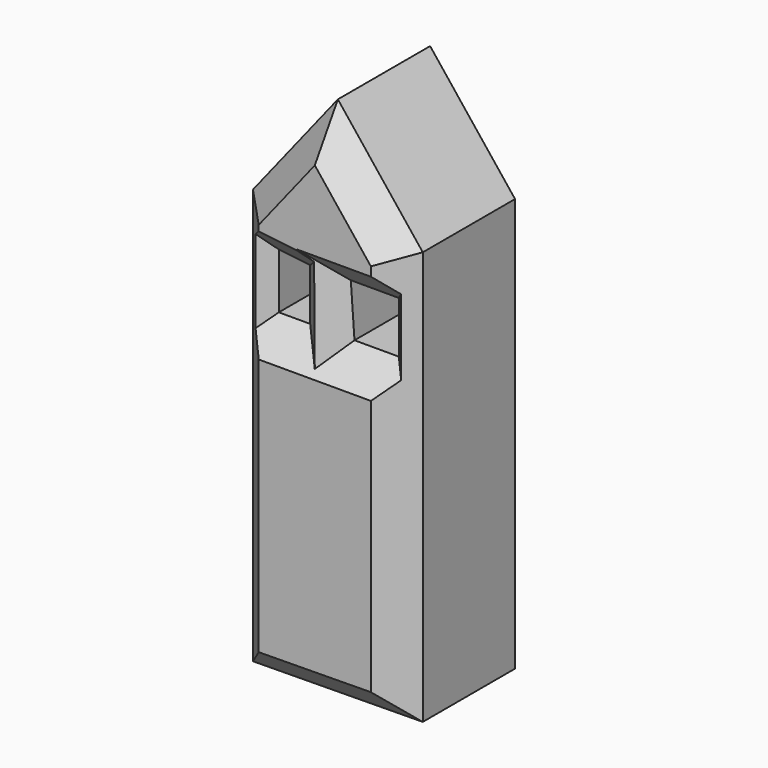
from build123d import *

# Parameters (mm, degrees)
F1_DEPTH      = 25.4
F2_T1_DEPTH   = 5.5291503668
F2_T3_DEPTH   = 9.1068297625
F2_T8_DEPTH   = 98.9829335321
F2_T14_DEPTH  = 50.2051374371
F2_T20_DEPTH  = 50.2051368583
F2_T26_DEPTH  = 99.3081774522
F2_T32_DEPTH  = 56.0525045898
F2_T38_DEPTH  = 22.8214690441
F2_T43_DEPTH  = 31.6955822143
F2_T49_DEPTH  = 22.1709793413
F2_T54_DEPTH  = 35.2583310718
F2_T60_DEPTH  = 21.5204924325
F2_T65_DEPTH  = 20.8700045923
F2_T71_DEPTH  = 98.9829335321
F2_T75_DEPTH  = 56.0525045898
F2_T82_DEPTH  = 98.9829335321
F2_T86_DEPTH  = 50.2051374371
F2_T93_DEPTH  = 50.2051374371
F2_T97_DEPTH  = 50.2051368583
F2_T104_DEPTH = 50.2051368583
F2_T108_DEPTH = 99.3081774522
F2_T115_DEPTH = 99.3081774522
F2_T119_DEPTH = 56.0525045898
F2_T126_DEPTH = 35.885618623
F2_T130_DEPTH = 18.5932999456
F2_T137_DEPTH = 22.8214690441
F2_T141_DEPTH = 31.6955822143
F2_T148_DEPTH = 31.6955822143
F2_T152_DEPTH = 22.1709793413
F2_T159_DEPTH = 35.2351289202
F2_T163_DEPTH = 18.5932999456
F2_T170_DEPTH = 35.2583310718
F2_T174_DEPTH = 20.8700045923
F2_T181_DEPTH = 35.2583310718
F2_T185_DEPTH = 21.5204924325
F2_T192_DEPTH = 34.5846420113
F2_T196_DEPTH = 22.1709793413
F2_T203_DEPTH = 22.1709793413
F2_T207_DEPTH = 33.9341541712
F3_R          = 2.4287646607
F4_DEPTH      = 25.4


# Not quite as in the source:
# - a fillet or chamfer that OpenCascade refuses, or shapes differently, is made with other operations: its cross-section is extruded or revolved along the edge and cut away or added


with BuildPart() as f1:
    # F0 (on Front) → F1 (new body)
    with BuildSketch(Plane.XZ):
        Polygon((-38.8666465878, 36.5899391472), (-38.8666465878, -36.5899391472), (-8.9442087337, -36.2646952271), (-8.9442087337, 36.5899391472), align=None)
        Polygon((-34.3132354319, 19.0267674625), (-34.3132354319, 28.7840869278), (-28.7840850651, 28.133597225), (-28.7840850651, 19.0267674625), align=None, mode=Mode.SUBTRACT)
        Polygon((-20.9782328457, 19.0267674625), (-21.6287206858, 28.133597225), (-13.1723778322, 28.133597225), (-13.1723778322, 19.0267674625), align=None, mode=Mode.SUBTRACT)
        Polygon((-23.9054281265, 55.4540865123), (-38.8666465878, 36.5899391472), (-8.9442087337, 36.5899391472), align=None)
    extrude(amount=F1_DEPTH)

    # F2: chamfer of 5.08 on 13 edges, made by hand

    # F2_s2 → F2_t1 (cut)
    with BuildSketch(Plane.YZ.offset(-34.3132354319)):
        with BuildLine():
            Line((-20.1763159021, 19.1704515604), (-25.5436840979, 13.8030833646))
            Line((-25.5436840979, 13.8030833646), (-25.6452840979, 13.8030833646))
            ThreePointArc((-25.6452840979, 13.8030833646), (-25.5016, 16.4149254135), (-25.5016, 19.0267674625))
            Line((-25.5016, 19.0267674625), (-25.4, 19.1283674625))
            ThreePointArc((-25.4, 19.1283674625), (-22.788157951, 19.1283674625), (-20.1763159021, 19.2720515604))
            Line((-20.1763159021, 19.2720515604), (-20.1763159021, 19.1704515604))
        make_face()
    extrude(amount=F2_T1_DEPTH, mode=Mode.SUBTRACT)

    # F2_s4 → F2_t3 (cut)
    with BuildSketch(Plane.XY.offset(19.0267674625)):
        with BuildLine():
            Line((-13.3160619302, -20.1763159021), (-7.9486937343, -25.5436840979))
            Line((-7.9486937343, -25.5436840979), (-7.9486937343, -25.6452840979))
            ThreePointArc((-7.9486937343, -25.6452840979), (-10.5605357833, -25.5016), (-13.1723778322, -25.5016))
            Line((-13.1723778322, -25.5016), (-13.2739778322, -25.4))
            ThreePointArc((-13.2739778322, -25.4), (-13.2739778322, -22.788157951), (-13.4176619302, -20.1763159021))
            Line((-13.4176619302, -20.1763159021), (-13.3160619302, -20.1763159021))
        make_face()
    extrude(amount=F2_T3_DEPTH, mode=Mode.SUBTRACT)


with BuildPart() as f2_tool6:
    # F2_s7 → F2_t8 (new body)
    with BuildSketch(Plane.XY.offset(-49.328844806)):
        with BuildLine():
            Line((-8.8005246358, -20.1763159021), (-14.1678928317, -25.5436840979))
            Line((-14.1678928317, -25.5436840979), (-14.1678928317, -25.6452840979))
            ThreePointArc((-14.1678928317, -25.6452840979), (-11.5560507827, -25.5016), (-8.9442087337, -25.5016))
            Line((-8.9442087337, -25.5016), (-8.8426087337, -25.4))
            ThreePointArc((-8.8426087337, -25.4), (-8.8426087337, -22.788157951), (-8.6989246358, -20.1763159021))
            Line((-8.6989246358, -20.1763159021), (-8.8005246358, -20.1763159021))
        make_face()
    extrude(amount=F2_T8_DEPTH)

    split(bisect_by=Plane(origin=(0.3930783298, 0, -36.163202967), x_dir=(0, 1, 0), z_dir=(-0.0108689242, 0, 0.9999409315)), keep=Keep.TOP)

    split(bisect_by=Plane(origin=(12.3236563201, 0, 9.7739337144), x_dir=(0, 1, 0), z_dir=(-0.7834976979, 0, -0.6213946873)), keep=Keep.TOP)


with BuildPart() as f1_1:
    add(f1.part)

    # F2_t5: cut F2_tool6
    add(f2_tool6.part, mode=Mode.SUBTRACT)


with BuildPart() as f2_tool12:
    # F2_s13 → F2_t14 (new body)
    with BuildSketch(Plane(origin=(-13.149871912, 0, 16.5802743125), x_dir=(0, 1, 0), z_dir=(-0.6213946873, 0, 0.7834976979))):
        with BuildLine():
            Line((-20.1763159021, -15.8727109385), (-25.5436840979, -10.5053427426))
            Line((-25.5436840979, -10.5053427426), (-25.6452840979, -10.5053427426))
            ThreePointArc((-25.6452840979, -10.5053427426), (-25.5016, -13.1171847916), (-25.5016, -15.7290268405))
            Line((-25.5016, -15.7290268405), (-25.4, -15.8306268405))
            ThreePointArc((-25.4, -15.8306268405), (-22.788157951, -15.8306268405), (-20.1763159021, -15.9743109385))
            Line((-20.1763159021, -15.9743109385), (-20.1763159021, -15.8727109385))
        make_face()
    extrude(amount=F2_T14_DEPTH)

    split(bisect_by=Plane.YZ.offset(-8.9442087337), keep=Keep.BOTTOM)

    split(bisect_by=Plane(origin=(-41.6732420747, 0, 33.0511878754), x_dir=(0, 1, 0), z_dir=(0.7834977168, 0, -0.6213946635)), keep=Keep.TOP)


with BuildPart() as f1_2:
    add(f1_1.part)

    # F2_t11: cut F2_tool12
    add(f2_tool12.part, mode=Mode.SUBTRACT)


with BuildPart() as f2_tool18:
    # F2_s19 → F2_t20 (new body)
    with BuildSketch(Plane(origin=(25.8858067798, 0, 32.6386300033), x_dir=(0, 1, 0), z_dir=(-0.6213946635, 0, -0.7834977168))):
        with BuildLine():
            Line((-20.1763159021, -53.3324058817), (-25.5436840979, -47.9650376858))
            Line((-25.5436840979, -47.9650376858), (-25.6452840979, -47.9650376858))
            ThreePointArc((-25.6452840979, -47.9650376858), (-25.5016, -50.5768797348), (-25.5016, -53.1887217838))
            Line((-25.5016, -53.1887217838), (-25.4, -53.2903217838))
            ThreePointArc((-25.4, -53.2903217838), (-22.788157951, -53.2903217838), (-20.1763159021, -53.4340058817))
            Line((-20.1763159021, -53.4340058817), (-20.1763159021, -53.3324058817))
        make_face()
    extrude(amount=F2_T20_DEPTH)

    split(bisect_by=Plane(origin=(12.3236563201, 0, 9.7739337144), x_dir=(0, 1, 0), z_dir=(-0.7834976979, 0, -0.6213946873)), keep=Keep.TOP)

    split(bisect_by=Plane.YZ.offset(-38.8666465878), keep=Keep.TOP)


with BuildPart() as f1_3:
    add(f1_2.part)

    # F2_t17: cut F2_tool18
    add(f2_tool18.part, mode=Mode.SUBTRACT)


with BuildPart() as f2_tool24:
    # F2_s25 → F2_t26 (new body)
    with BuildSketch(Plane.XY.offset(49.6540887261)):
        with BuildLine():
            Line((-39.0103306858, -20.1763159021), (-33.6429624899, -25.5436840979))
            Line((-33.6429624899, -25.5436840979), (-33.6429624899, -25.6452840979))
            ThreePointArc((-33.6429624899, -25.6452840979), (-36.2548045389, -25.5016), (-38.8666465878, -25.5016))
            Line((-38.8666465878, -25.5016), (-38.9682465878, -25.4))
            ThreePointArc((-38.9682465878, -25.4), (-38.9682465878, -22.788157951), (-39.1119306858, -20.1763159021))
            Line((-39.1119306858, -20.1763159021), (-39.0103306858, -20.1763159021))
        make_face()
    extrude(amount=-F2_T26_DEPTH)

    split(bisect_by=Plane(origin=(-41.6732420747, 0, 33.0511878754), x_dir=(0, 1, 0), z_dir=(0.7834977168, 0, -0.6213946635)), keep=Keep.TOP)

    split(bisect_by=Plane(origin=(0.3930783298, 0, -36.163202967), x_dir=(0, 1, 0), z_dir=(-0.0108689242, 0, 0.9999409315)), keep=Keep.TOP)


with BuildPart() as f1_4:
    add(f1_3.part)

    # F2_t23: cut F2_tool24
    add(f2_tool24.part, mode=Mode.SUBTRACT)


with BuildPart() as f2_tool30:
    # F2_s31 → F2_t32 (new body)
    with BuildSketch(Plane(origin=(-52.3231028168, 0, -0.5687294315), x_dir=(0, 1, 0), z_dir=(0.9999409315, 0, 0.0108689242))):
        with BuildLine():
            Line((-20.1763159021, -36.3090232973), (-25.5436840979, -30.9416551014))
            Line((-25.5436840979, -30.9416551014), (-25.6452840979, -30.9416551014))
            ThreePointArc((-25.6452840979, -30.9416551014), (-25.5016, -33.5534971504), (-25.5016, -36.1653391994))
            Line((-25.5016, -36.1653391994), (-25.4, -36.2669391994))
            ThreePointArc((-25.4, -36.2669391994), (-22.788157951, -36.2669391994), (-20.1763159021, -36.4106232973))
            Line((-20.1763159021, -36.4106232973), (-20.1763159021, -36.3090232973))
        make_face()
    extrude(amount=F2_T32_DEPTH)

    split(bisect_by=Plane.YZ.offset(-8.9442087337), keep=Keep.BOTTOM)

    split(bisect_by=Plane.YZ.offset(-38.8666465878), keep=Keep.TOP)


with BuildPart() as f1_5:
    add(f1_4.part)

    # F2_t29: cut F2_tool30
    add(f2_tool30.part, mode=Mode.SUBTRACT)


with BuildPart() as f2_tool36:
    # F2_s37 → F2_t38 (new body)
    with BuildSketch(Plane.XY.offset(19.0267674625)):
        with BuildLine():
            Line((-34.169551334, -20.1763159021), (-39.5369195298, -25.5436840979))
            Line((-39.5369195298, -25.5436840979), (-39.5369195298, -25.6452840979))
            ThreePointArc((-39.5369195298, -25.6452840979), (-36.9250774809, -25.5016), (-34.3132354319, -25.5016))
            Line((-34.3132354319, -25.5016), (-34.2116354319, -25.4))
            ThreePointArc((-34.2116354319, -25.4), (-34.2116354319, -22.788157951), (-34.067951334, -20.1763159021))
            Line((-34.067951334, -20.1763159021), (-34.169551334, -20.1763159021))
        make_face()
    extrude(amount=F2_T38_DEPTH)

    split(bisect_by=Plane(origin=(2.8716979706, 0, 24.4093793011), x_dir=(0, 1, 0), z_dir=(-0.1168414999, 0, -0.9931505746)), keep=Keep.TOP)


with BuildPart() as f1_6:
    add(f1_5.part)

    # F2_t35: cut F2_tool36
    add(f2_tool36.part, mode=Mode.SUBTRACT)


with BuildPart() as f2_tool41:
    # F2_s42 → F2_t43 (new body)
    with BuildSketch(Plane(origin=(-50.1596010639, 0, 5.9011424586), x_dir=(0, 1, 0), z_dir=(0.9931505746, 0, -0.1168414999))):
        with BuildLine():
            Line((-20.1763159021, 24.4340384796), (-25.5436840979, 29.8014066755))
            Line((-25.5436840979, 29.8014066755), (-25.6452840979, 29.8014066755))
            ThreePointArc((-25.6452840979, 29.8014066755), (-25.5016, 27.1895646266), (-25.5016, 24.5777225776))
            Line((-25.5016, 24.5777225776), (-25.4, 24.4761225776))
            ThreePointArc((-25.4, 24.4761225776), (-22.788157951, 24.4761225776), (-20.1763159021, 24.3324384796))
            Line((-20.1763159021, 24.3324384796), (-20.1763159021, 24.4340384796))
        make_face()
    extrude(amount=F2_T43_DEPTH)

    split(bisect_by=Plane.YZ.offset(-34.3132354319), keep=Keep.TOP)

    split(bisect_by=Plane.YZ.offset(-28.7840850651), keep=Keep.BOTTOM)


with BuildPart() as f1_7:
    add(f1_6.part)

    # F2_t40: cut F2_tool41
    add(f2_tool41.part, mode=Mode.SUBTRACT)


with BuildPart() as f2_tool47:
    # F2_s48 → F2_t49 (new body)
    with BuildSketch(Plane.XY.offset(41.1977468038)):
        with BuildLine():
            Line((-28.9277691631, -20.1763159021), (-23.5604009672, -25.5436840979))
            Line((-23.5604009672, -25.5436840979), (-23.5604009672, -25.6452840979))
            ThreePointArc((-23.5604009672, -25.6452840979), (-26.1722430162, -25.5016), (-28.7840850651, -25.5016))
            Line((-28.7840850651, -25.5016), (-28.8856850651, -25.4))
            ThreePointArc((-28.8856850651, -25.4), (-28.8856850651, -22.788157951), (-29.0293691631, -20.1763159021))
            Line((-29.0293691631, -20.1763159021), (-28.9277691631, -20.1763159021))
        make_face()
    extrude(amount=-F2_T49_DEPTH)

    split(bisect_by=Plane(origin=(2.8716979706, 0, 24.4093793011), x_dir=(0, 1, 0), z_dir=(-0.1168414999, 0, -0.9931505746)), keep=Keep.TOP)


with BuildPart() as f1_8:
    add(f1_7.part)

    # F2_t46: cut F2_tool47
    add(f2_tool47.part, mode=Mode.SUBTRACT)


with BuildPart() as f2_tool52:
    # F2_s53 → F2_t54 (new body)
    with BuildSketch(Plane(origin=(-0.5278624368, 0, 7.3900741156), x_dir=(0, 1, 0), z_dir=(-0.07124705, 0, 0.9974586998))):
        with BuildLine():
            Line((-20.1763159021, 19.4256357085), (-25.5436840979, 24.7930039044))
            Line((-25.5436840979, 24.7930039044), (-25.6452840979, 24.7930039044))
            ThreePointArc((-25.6452840979, 24.7930039044), (-25.5016, 22.1811618554), (-25.5016, 19.5693198065))
            Line((-25.5016, 19.5693198065), (-25.4, 19.4677198065))
            ThreePointArc((-25.4, 19.4677198065), (-22.788157951, 19.4677198065), (-20.1763159021, 19.3240357085))
            Line((-20.1763159021, 19.3240357085), (-20.1763159021, 19.4256357085))
        make_face()
    extrude(amount=F2_T54_DEPTH)

    split(bisect_by=Plane.XY.offset(19.0267674625), keep=Keep.TOP)

    split(bisect_by=Plane.XY.offset(28.133597225), keep=Keep.BOTTOM)


with BuildPart() as f1_9:
    add(f1_8.part)

    # F2_t51: cut F2_tool52
    add(f2_tool52.part, mode=Mode.SUBTRACT)


with BuildPart() as f2_tool58:
    # F2_s59 → F2_t60 (new body)
    with BuildSketch(Plane.YZ.offset(-34.6928702647)):
        with BuildLine():
            Line((-20.1763159021, 27.989913127), (-25.5436840979, 33.3572813229))
            Line((-25.5436840979, 33.3572813229), (-25.6452840979, 33.3572813229))
            ThreePointArc((-25.6452840979, 33.3572813229), (-25.5016, 30.7454392739), (-25.5016, 28.133597225))
            Line((-25.5016, 28.133597225), (-25.4, 28.031997225))
            ThreePointArc((-25.4, 28.031997225), (-22.788157951, 28.031997225), (-20.1763159021, 27.888313127))
            Line((-20.1763159021, 27.888313127), (-20.1763159021, 27.989913127))
        make_face()
    extrude(amount=F2_T60_DEPTH)

    split(bisect_by=Plane(origin=(-19.5195882907, 0, -1.3942563065), x_dir=(0, 1, 0), z_dir=(0.9974586998, 0, 0.07124705)), keep=Keep.TOP)


with BuildPart() as f1_10:
    add(f1_9.part)

    # F2_t57: cut F2_tool58
    add(f2_tool58.part, mode=Mode.SUBTRACT)


with BuildPart() as f2_tool63:
    # F2_s64 → F2_t65 (new body)
    with BuildSketch(Plane.YZ.offset(-13.1723778322)):
        with BuildLine():
            Line((-20.1763159021, 19.1704515604), (-25.5436840979, 13.8030833646))
            Line((-25.5436840979, 13.8030833646), (-25.6452840979, 13.8030833646))
            ThreePointArc((-25.6452840979, 13.8030833646), (-25.5016, 16.4149254135), (-25.5016, 19.0267674625))
            Line((-25.5016, 19.0267674625), (-25.4, 19.1283674625))
            ThreePointArc((-25.4, 19.1283674625), (-22.788157951, 19.1283674625), (-20.1763159021, 19.2720515604))
            Line((-20.1763159021, 19.2720515604), (-20.1763159021, 19.1704515604))
        make_face()
    extrude(amount=-F2_T65_DEPTH)

    split(bisect_by=Plane(origin=(-19.5195882907, 0, -1.3942563065), x_dir=(0, 1, 0), z_dir=(0.9974586998, 0, 0.07124705)), keep=Keep.TOP)


with BuildPart() as f1_11:
    add(f1_10.part)

    # F2_t62: cut F2_tool63
    add(f2_tool63.part, mode=Mode.SUBTRACT)


with BuildPart() as f2_tool69:
    # F2_s70 → F2_t71 (new body)
    with BuildSketch(Plane.XY.offset(-49.328844806)):
        with BuildLine():
            Line((-8.8005246358, -20.1763159021), (-14.1678928317, -25.5436840979))
            Line((-14.1678928317, -25.5436840979), (-14.1678928317, -25.6452840979))
            ThreePointArc((-14.1678928317, -25.6452840979), (-11.5560507827, -25.5016), (-8.9442087337, -25.5016))
            Line((-8.9442087337, -25.5016), (-8.8426087337, -25.4))
            ThreePointArc((-8.8426087337, -25.4), (-8.8426087337, -22.788157951), (-8.6989246358, -20.1763159021))
            Line((-8.6989246358, -20.1763159021), (-8.8005246358, -20.1763159021))
        make_face()
    extrude(amount=F2_T71_DEPTH)

    split(bisect_by=Plane(origin=(0.3930783298, 0, -36.163202967), x_dir=(0, 1, 0), z_dir=(0.0108689242, 0, -0.9999409315)), keep=Keep.TOP)


with BuildPart() as f2_tool73:
    # F2_s74 → F2_t75 (new body)
    with BuildSketch(Plane(origin=(-52.3231028168, 0, -0.5687294315), x_dir=(0, 1, 0), z_dir=(0.9999409315, 0, 0.0108689242))):
        with BuildLine():
            Line((-20.1763159021, -36.3090232973), (-25.5436840979, -30.9416551014))
            Line((-25.5436840979, -30.9416551014), (-25.6452840979, -30.9416551014))
            ThreePointArc((-25.6452840979, -30.9416551014), (-25.5016, -33.5534971504), (-25.5016, -36.1653391994))
            Line((-25.5016, -36.1653391994), (-25.4, -36.2669391994))
            ThreePointArc((-25.4, -36.2669391994), (-22.788157951, -36.2669391994), (-20.1763159021, -36.4106232973))
            Line((-20.1763159021, -36.4106232973), (-20.1763159021, -36.3090232973))
        make_face()
    extrude(amount=F2_T75_DEPTH)

    split(bisect_by=Plane.YZ.offset(-8.9442087337), keep=Keep.TOP)


with BuildPart() as f2_tool69_1:
    add(f2_tool69.part)

    # F2_t77: intersect F2_tool73
    add(f2_tool73.part, mode=Mode.INTERSECT)


with BuildPart() as f1_12:
    add(f1_11.part)

    # F2_t67: cut F2_tool69
    add(f2_tool69_1.part, mode=Mode.SUBTRACT)


with BuildPart() as f2_tool80:
    # F2_s81 → F2_t82 (new body)
    with BuildSketch(Plane.XY.offset(-49.328844806)):
        with BuildLine():
            Line((-8.8005246358, -20.1763159021), (-14.1678928317, -25.5436840979))
            Line((-14.1678928317, -25.5436840979), (-14.1678928317, -25.6452840979))
            ThreePointArc((-14.1678928317, -25.6452840979), (-11.5560507827, -25.5016), (-8.9442087337, -25.5016))
            Line((-8.9442087337, -25.5016), (-8.8426087337, -25.4))
            ThreePointArc((-8.8426087337, -25.4), (-8.8426087337, -22.788157951), (-8.6989246358, -20.1763159021))
            Line((-8.6989246358, -20.1763159021), (-8.8005246358, -20.1763159021))
        make_face()
    extrude(amount=F2_T82_DEPTH)

    split(bisect_by=Plane(origin=(12.3236563201, 0, 9.7739337144), x_dir=(0, 1, 0), z_dir=(0.7834976979, 0, 0.6213946873)), keep=Keep.TOP)


with BuildPart() as f2_tool84:
    # F2_s85 → F2_t86 (new body)
    with BuildSketch(Plane(origin=(-13.149871912, 0, 16.5802743125), x_dir=(0, 1, 0), z_dir=(-0.6213946873, 0, 0.7834976979))):
        with BuildLine():
            Line((-20.1763159021, -15.8727109385), (-25.5436840979, -10.5053427426))
            Line((-25.5436840979, -10.5053427426), (-25.6452840979, -10.5053427426))
            ThreePointArc((-25.6452840979, -10.5053427426), (-25.5016, -13.1171847916), (-25.5016, -15.7290268405))
            Line((-25.5016, -15.7290268405), (-25.4, -15.8306268405))
            ThreePointArc((-25.4, -15.8306268405), (-22.788157951, -15.8306268405), (-20.1763159021, -15.9743109385))
            Line((-20.1763159021, -15.9743109385), (-20.1763159021, -15.8727109385))
        make_face()
    extrude(amount=F2_T86_DEPTH)

    split(bisect_by=Plane.YZ.offset(-8.9442087337), keep=Keep.TOP)


with BuildPart() as f2_tool80_1:
    add(f2_tool80.part)

    # F2_t88: intersect F2_tool84
    add(f2_tool84.part, mode=Mode.INTERSECT)


with BuildPart() as f1_13:
    add(f1_12.part)

    # F2_t78: cut F2_tool80
    add(f2_tool80_1.part, mode=Mode.SUBTRACT)


with BuildPart() as f2_tool91:
    # F2_s92 → F2_t93 (new body)
    with BuildSketch(Plane(origin=(-13.149871912, 0, 16.5802743125), x_dir=(0, 1, 0), z_dir=(-0.6213946873, 0, 0.7834976979))):
        with BuildLine():
            Line((-20.1763159021, -15.8727109385), (-25.5436840979, -10.5053427426))
            Line((-25.5436840979, -10.5053427426), (-25.6452840979, -10.5053427426))
            ThreePointArc((-25.6452840979, -10.5053427426), (-25.5016, -13.1171847916), (-25.5016, -15.7290268405))
            Line((-25.5016, -15.7290268405), (-25.4, -15.8306268405))
            ThreePointArc((-25.4, -15.8306268405), (-22.788157951, -15.8306268405), (-20.1763159021, -15.9743109385))
            Line((-20.1763159021, -15.9743109385), (-20.1763159021, -15.8727109385))
        make_face()
    extrude(amount=F2_T93_DEPTH)

    split(bisect_by=Plane(origin=(-41.6732420747, 0, 33.0511878754), x_dir=(0, 1, 0), z_dir=(-0.7834977168, 0, 0.6213946635)), keep=Keep.TOP)


with BuildPart() as f2_tool95:
    # F2_s96 → F2_t97 (new body)
    with BuildSketch(Plane(origin=(25.8858067798, 0, 32.6386300033), x_dir=(0, 1, 0), z_dir=(-0.6213946635, 0, -0.7834977168))):
        with BuildLine():
            Line((-20.1763159021, -53.3324058817), (-25.5436840979, -47.9650376858))
            Line((-25.5436840979, -47.9650376858), (-25.6452840979, -47.9650376858))
            ThreePointArc((-25.6452840979, -47.9650376858), (-25.5016, -50.5768797348), (-25.5016, -53.1887217838))
            Line((-25.5016, -53.1887217838), (-25.4, -53.2903217838))
            ThreePointArc((-25.4, -53.2903217838), (-22.788157951, -53.2903217838), (-20.1763159021, -53.4340058817))
            Line((-20.1763159021, -53.4340058817), (-20.1763159021, -53.3324058817))
        make_face()
    extrude(amount=F2_T97_DEPTH)

    split(bisect_by=Plane(origin=(12.3236563201, 0, 9.7739337144), x_dir=(0, 1, 0), z_dir=(0.7834976979, 0, 0.6213946873)), keep=Keep.TOP)


with BuildPart() as f2_tool91_1:
    add(f2_tool91.part)

    # F2_t99: intersect F2_tool95
    add(f2_tool95.part, mode=Mode.INTERSECT)


with BuildPart() as f1_14:
    add(f1_13.part)

    # F2_t89: cut F2_tool91
    add(f2_tool91_1.part, mode=Mode.SUBTRACT)


with BuildPart() as f2_tool102:
    # F2_s103 → F2_t104 (new body)
    with BuildSketch(Plane(origin=(25.8858067798, 0, 32.6386300033), x_dir=(0, 1, 0), z_dir=(-0.6213946635, 0, -0.7834977168))):
        with BuildLine():
            Line((-20.1763159021, -53.3324058817), (-25.5436840979, -47.9650376858))
            Line((-25.5436840979, -47.9650376858), (-25.6452840979, -47.9650376858))
            ThreePointArc((-25.6452840979, -47.9650376858), (-25.5016, -50.5768797348), (-25.5016, -53.1887217838))
            Line((-25.5016, -53.1887217838), (-25.4, -53.2903217838))
            ThreePointArc((-25.4, -53.2903217838), (-22.788157951, -53.2903217838), (-20.1763159021, -53.4340058817))
            Line((-20.1763159021, -53.4340058817), (-20.1763159021, -53.3324058817))
        make_face()
    extrude(amount=F2_T104_DEPTH)

    split(bisect_by=Plane.YZ.offset(-38.8666465878), keep=Keep.BOTTOM)


with BuildPart() as f2_tool106:
    # F2_s107 → F2_t108 (new body)
    with BuildSketch(Plane.XY.offset(49.6540887261)):
        with BuildLine():
            Line((-39.0103306858, -20.1763159021), (-33.6429624899, -25.5436840979))
            Line((-33.6429624899, -25.5436840979), (-33.6429624899, -25.6452840979))
            ThreePointArc((-33.6429624899, -25.6452840979), (-36.2548045389, -25.5016), (-38.8666465878, -25.5016))
            Line((-38.8666465878, -25.5016), (-38.9682465878, -25.4))
            ThreePointArc((-38.9682465878, -25.4), (-38.9682465878, -22.788157951), (-39.1119306858, -20.1763159021))
            Line((-39.1119306858, -20.1763159021), (-39.0103306858, -20.1763159021))
        make_face()
    extrude(amount=-F2_T108_DEPTH)

    split(bisect_by=Plane(origin=(-41.6732420747, 0, 33.0511878754), x_dir=(0, 1, 0), z_dir=(-0.7834977168, 0, 0.6213946635)), keep=Keep.TOP)


with BuildPart() as f2_tool102_1:
    add(f2_tool102.part)

    # F2_t110: intersect F2_tool106
    add(f2_tool106.part, mode=Mode.INTERSECT)


with BuildPart() as f1_15:
    add(f1_14.part)

    # F2_t100: cut F2_tool102
    add(f2_tool102_1.part, mode=Mode.SUBTRACT)


with BuildPart() as f2_tool113:
    # F2_s114 → F2_t115 (new body)
    with BuildSketch(Plane.XY.offset(49.6540887261)):
        with BuildLine():
            Line((-39.0103306858, -20.1763159021), (-33.6429624899, -25.5436840979))
            Line((-33.6429624899, -25.5436840979), (-33.6429624899, -25.6452840979))
            ThreePointArc((-33.6429624899, -25.6452840979), (-36.2548045389, -25.5016), (-38.8666465878, -25.5016))
            Line((-38.8666465878, -25.5016), (-38.9682465878, -25.4))
            ThreePointArc((-38.9682465878, -25.4), (-38.9682465878, -22.788157951), (-39.1119306858, -20.1763159021))
            Line((-39.1119306858, -20.1763159021), (-39.0103306858, -20.1763159021))
        make_face()
    extrude(amount=-F2_T115_DEPTH)

    split(bisect_by=Plane(origin=(0.3930783298, 0, -36.163202967), x_dir=(0, 1, 0), z_dir=(0.0108689242, 0, -0.9999409315)), keep=Keep.TOP)


with BuildPart() as f2_tool117:
    # F2_s118 → F2_t119 (new body)
    with BuildSketch(Plane(origin=(-52.3231028168, 0, -0.5687294315), x_dir=(0, 1, 0), z_dir=(0.9999409315, 0, 0.0108689242))):
        with BuildLine():
            Line((-20.1763159021, -36.3090232973), (-25.5436840979, -30.9416551014))
            Line((-25.5436840979, -30.9416551014), (-25.6452840979, -30.9416551014))
            ThreePointArc((-25.6452840979, -30.9416551014), (-25.5016, -33.5534971504), (-25.5016, -36.1653391994))
            Line((-25.5016, -36.1653391994), (-25.4, -36.2669391994))
            ThreePointArc((-25.4, -36.2669391994), (-22.788157951, -36.2669391994), (-20.1763159021, -36.4106232973))
            Line((-20.1763159021, -36.4106232973), (-20.1763159021, -36.3090232973))
        make_face()
    extrude(amount=F2_T119_DEPTH)

    split(bisect_by=Plane.YZ.offset(-38.8666465878), keep=Keep.BOTTOM)


with BuildPart() as f2_tool113_1:
    add(f2_tool113.part)

    # F2_t121: intersect F2_tool117
    add(f2_tool117.part, mode=Mode.INTERSECT)


with BuildPart() as f1_16:
    add(f1_15.part)

    # F2_t111: cut F2_tool113
    add(f2_tool113_1.part, mode=Mode.SUBTRACT)


with BuildPart() as f2_tool124:
    # F2_s125 → F2_t126 (new body)
    with BuildSketch(Plane.XY.offset(5.9626178836)):
        with BuildLine():
            Line((-34.169551334, -20.1763159021), (-39.5369195298, -25.5436840979))
            Line((-39.5369195298, -25.5436840979), (-39.5369195298, -25.6452840979))
            ThreePointArc((-39.5369195298, -25.6452840979), (-36.9250774809, -25.5016), (-34.3132354319, -25.5016))
            Line((-34.3132354319, -25.5016), (-34.2116354319, -25.4))
            ThreePointArc((-34.2116354319, -25.4), (-34.2116354319, -22.788157951), (-34.067951334, -20.1763159021))
            Line((-34.067951334, -20.1763159021), (-34.169551334, -20.1763159021))
        make_face()
    extrude(amount=F2_T126_DEPTH)

    split(bisect_by=Plane.XY.offset(19.0267674625), keep=Keep.BOTTOM)


with BuildPart() as f2_tool128:
    # F2_s129 → F2_t130 (new body)
    with BuildSketch(Plane.YZ.offset(-28.7840850651)):
        with BuildLine():
            Line((-20.1763159021, 19.1704515604), (-25.5436840979, 13.8030833646))
            Line((-25.5436840979, 13.8030833646), (-25.6452840979, 13.8030833646))
            ThreePointArc((-25.6452840979, 13.8030833646), (-25.5016, 16.4149254135), (-25.5016, 19.0267674625))
            Line((-25.5016, 19.0267674625), (-25.4, 19.1283674625))
            ThreePointArc((-25.4, 19.1283674625), (-22.788157951, 19.1283674625), (-20.1763159021, 19.2720515604))
            Line((-20.1763159021, 19.2720515604), (-20.1763159021, 19.1704515604))
        make_face()
    extrude(amount=-F2_T130_DEPTH)

    split(bisect_by=Plane.YZ.offset(-34.3132354319), keep=Keep.BOTTOM)


with BuildPart() as f2_tool124_1:
    add(f2_tool124.part)

    # F2_t132: intersect F2_tool128
    add(f2_tool128.part, mode=Mode.INTERSECT)


with BuildPart() as f1_17:
    add(f1_16.part)

    # F2_t122: cut F2_tool124
    add(f2_tool124_1.part, mode=Mode.SUBTRACT)


with BuildPart() as f2_tool135:
    # F2_s136 → F2_t137 (new body)
    with BuildSketch(Plane.XY.offset(19.0267674625)):
        with BuildLine():
            Line((-34.169551334, -20.1763159021), (-39.5369195298, -25.5436840979))
            Line((-39.5369195298, -25.5436840979), (-39.5369195298, -25.6452840979))
            ThreePointArc((-39.5369195298, -25.6452840979), (-36.9250774809, -25.5016), (-34.3132354319, -25.5016))
            Line((-34.3132354319, -25.5016), (-34.2116354319, -25.4))
            ThreePointArc((-34.2116354319, -25.4), (-34.2116354319, -22.788157951), (-34.067951334, -20.1763159021))
            Line((-34.067951334, -20.1763159021), (-34.169551334, -20.1763159021))
        make_face()
    extrude(amount=F2_T137_DEPTH)

    split(bisect_by=Plane(origin=(2.8716979706, 0, 24.4093793011), x_dir=(0, 1, 0), z_dir=(0.1168414999, 0, 0.9931505746)), keep=Keep.TOP)


with BuildPart() as f2_tool139:
    # F2_s140 → F2_t141 (new body)
    with BuildSketch(Plane(origin=(-50.1596010639, 0, 5.9011424586), x_dir=(0, 1, 0), z_dir=(0.9931505746, 0, -0.1168414999))):
        with BuildLine():
            Line((-20.1763159021, 24.4340384796), (-25.5436840979, 29.8014066755))
            Line((-25.5436840979, 29.8014066755), (-25.6452840979, 29.8014066755))
            ThreePointArc((-25.6452840979, 29.8014066755), (-25.5016, 27.1895646266), (-25.5016, 24.5777225776))
            Line((-25.5016, 24.5777225776), (-25.4, 24.4761225776))
            ThreePointArc((-25.4, 24.4761225776), (-22.788157951, 24.4761225776), (-20.1763159021, 24.3324384796))
            Line((-20.1763159021, 24.3324384796), (-20.1763159021, 24.4340384796))
        make_face()
    extrude(amount=F2_T141_DEPTH)

    split(bisect_by=Plane.YZ.offset(-34.3132354319), keep=Keep.BOTTOM)


with BuildPart() as f2_tool135_1:
    add(f2_tool135.part)

    # F2_t143: intersect F2_tool139
    add(f2_tool139.part, mode=Mode.INTERSECT)


with BuildPart() as f1_18:
    add(f1_17.part)

    # F2_t133: cut F2_tool135
    add(f2_tool135_1.part, mode=Mode.SUBTRACT)


with BuildPart() as f2_tool146:
    # F2_s147 → F2_t148 (new body)
    with BuildSketch(Plane(origin=(-50.1596010639, 0, 5.9011424586), x_dir=(0, 1, 0), z_dir=(0.9931505746, 0, -0.1168414999))):
        with BuildLine():
            Line((-20.1763159021, 24.4340384796), (-25.5436840979, 29.8014066755))
            Line((-25.5436840979, 29.8014066755), (-25.6452840979, 29.8014066755))
            ThreePointArc((-25.6452840979, 29.8014066755), (-25.5016, 27.1895646266), (-25.5016, 24.5777225776))
            Line((-25.5016, 24.5777225776), (-25.4, 24.4761225776))
            ThreePointArc((-25.4, 24.4761225776), (-22.788157951, 24.4761225776), (-20.1763159021, 24.3324384796))
            Line((-20.1763159021, 24.3324384796), (-20.1763159021, 24.4340384796))
        make_face()
    extrude(amount=F2_T148_DEPTH)

    split(bisect_by=Plane.YZ.offset(-28.7840850651), keep=Keep.TOP)


with BuildPart() as f2_tool150:
    # F2_s151 → F2_t152 (new body)
    with BuildSketch(Plane.XY.offset(41.1977468038)):
        with BuildLine():
            Line((-28.9277691631, -20.1763159021), (-23.5604009672, -25.5436840979))
            Line((-23.5604009672, -25.5436840979), (-23.5604009672, -25.6452840979))
            ThreePointArc((-23.5604009672, -25.6452840979), (-26.1722430162, -25.5016), (-28.7840850651, -25.5016))
            Line((-28.7840850651, -25.5016), (-28.8856850651, -25.4))
            ThreePointArc((-28.8856850651, -25.4), (-28.8856850651, -22.788157951), (-29.0293691631, -20.1763159021))
            Line((-29.0293691631, -20.1763159021), (-28.9277691631, -20.1763159021))
        make_face()
    extrude(amount=-F2_T152_DEPTH)

    split(bisect_by=Plane(origin=(2.8716979706, 0, 24.4093793011), x_dir=(0, 1, 0), z_dir=(0.1168414999, 0, 0.9931505746)), keep=Keep.TOP)


with BuildPart() as f2_tool146_1:
    add(f2_tool146.part)

    # F2_t154: intersect F2_tool150
    add(f2_tool150.part, mode=Mode.INTERSECT)


with BuildPart() as f1_19:
    add(f1_18.part)

    # F2_t144: cut F2_tool146
    add(f2_tool146_1.part, mode=Mode.SUBTRACT)


with BuildPart() as f2_tool157:
    # F2_s158 → F2_t159 (new body)
    with BuildSketch(Plane.XY.offset(41.1977468038)):
        with BuildLine():
            Line((-28.9277691631, -20.1763159021), (-23.5604009672, -25.5436840979))
            Line((-23.5604009672, -25.5436840979), (-23.5604009672, -25.6452840979))
            ThreePointArc((-23.5604009672, -25.6452840979), (-26.1722430162, -25.5016), (-28.7840850651, -25.5016))
            Line((-28.7840850651, -25.5016), (-28.8856850651, -25.4))
            ThreePointArc((-28.8856850651, -25.4), (-28.8856850651, -22.788157951), (-29.0293691631, -20.1763159021))
            Line((-29.0293691631, -20.1763159021), (-28.9277691631, -20.1763159021))
        make_face()
    extrude(amount=-F2_T159_DEPTH)

    split(bisect_by=Plane.XY.offset(19.0267674625), keep=Keep.BOTTOM)


with BuildPart() as f2_tool161:
    # F2_s162 → F2_t163 (new body)
    with BuildSketch(Plane.YZ.offset(-15.7199354863)):
        with BuildLine():
            Line((-20.1763159021, 19.1704515604), (-25.5436840979, 13.8030833646))
            Line((-25.5436840979, 13.8030833646), (-25.6452840979, 13.8030833646))
            ThreePointArc((-25.6452840979, 13.8030833646), (-25.5016, 16.4149254135), (-25.5016, 19.0267674625))
            Line((-25.5016, 19.0267674625), (-25.4, 19.1283674625))
            ThreePointArc((-25.4, 19.1283674625), (-22.788157951, 19.1283674625), (-20.1763159021, 19.2720515604))
            Line((-20.1763159021, 19.2720515604), (-20.1763159021, 19.1704515604))
        make_face()
    extrude(amount=-F2_T163_DEPTH)

    split(bisect_by=Plane.YZ.offset(-28.7840850651), keep=Keep.TOP)


with BuildPart() as f2_tool157_1:
    add(f2_tool157.part)

    # F2_t165: intersect F2_tool161
    add(f2_tool161.part, mode=Mode.INTERSECT)


with BuildPart() as f1_20:
    add(f1_19.part)

    # F2_t155: cut F2_tool157
    add(f2_tool157_1.part, mode=Mode.SUBTRACT)


with BuildPart() as f2_tool168:
    # F2_s169 → F2_t170 (new body)
    with BuildSketch(Plane(origin=(-0.5278624368, 0, 7.3900741156), x_dir=(0, 1, 0), z_dir=(-0.07124705, 0, 0.9974586998))):
        with BuildLine():
            Line((-20.1763159021, 19.4256357085), (-25.5436840979, 24.7930039044))
            Line((-25.5436840979, 24.7930039044), (-25.6452840979, 24.7930039044))
            ThreePointArc((-25.6452840979, 24.7930039044), (-25.5016, 22.1811618554), (-25.5016, 19.5693198065))
            Line((-25.5016, 19.5693198065), (-25.4, 19.4677198065))
            ThreePointArc((-25.4, 19.4677198065), (-22.788157951, 19.4677198065), (-20.1763159021, 19.3240357085))
            Line((-20.1763159021, 19.3240357085), (-20.1763159021, 19.4256357085))
        make_face()
    extrude(amount=F2_T170_DEPTH)

    split(bisect_by=Plane.XY.offset(19.0267674625), keep=Keep.BOTTOM)


with BuildPart() as f2_tool172:
    # F2_s173 → F2_t174 (new body)
    with BuildSketch(Plane.YZ.offset(-13.1723778322)):
        with BuildLine():
            Line((-20.1763159021, 19.1704515604), (-25.5436840979, 13.8030833646))
            Line((-25.5436840979, 13.8030833646), (-25.6452840979, 13.8030833646))
            ThreePointArc((-25.6452840979, 13.8030833646), (-25.5016, 16.4149254135), (-25.5016, 19.0267674625))
            Line((-25.5016, 19.0267674625), (-25.4, 19.1283674625))
            ThreePointArc((-25.4, 19.1283674625), (-22.788157951, 19.1283674625), (-20.1763159021, 19.2720515604))
            Line((-20.1763159021, 19.2720515604), (-20.1763159021, 19.1704515604))
        make_face()
    extrude(amount=-F2_T174_DEPTH)

    split(bisect_by=Plane(origin=(-19.5195882907, 0, -1.3942563065), x_dir=(0, 1, 0), z_dir=(-0.9974586998, 0, -0.07124705)), keep=Keep.TOP)


with BuildPart() as f2_tool168_1:
    add(f2_tool168.part)

    # F2_t176: intersect F2_tool172
    add(f2_tool172.part, mode=Mode.INTERSECT)


with BuildPart() as f1_21:
    add(f1_20.part)

    # F2_t166: cut F2_tool168
    add(f2_tool168_1.part, mode=Mode.SUBTRACT)


with BuildPart() as f2_tool179:
    # F2_s180 → F2_t181 (new body)
    with BuildSketch(Plane(origin=(-0.5278624368, 0, 7.3900741156), x_dir=(0, 1, 0), z_dir=(-0.07124705, 0, 0.9974586998))):
        with BuildLine():
            Line((-20.1763159021, 19.4256357085), (-25.5436840979, 24.7930039044))
            Line((-25.5436840979, 24.7930039044), (-25.6452840979, 24.7930039044))
            ThreePointArc((-25.6452840979, 24.7930039044), (-25.5016, 22.1811618554), (-25.5016, 19.5693198065))
            Line((-25.5016, 19.5693198065), (-25.4, 19.4677198065))
            ThreePointArc((-25.4, 19.4677198065), (-22.788157951, 19.4677198065), (-20.1763159021, 19.3240357085))
            Line((-20.1763159021, 19.3240357085), (-20.1763159021, 19.4256357085))
        make_face()
    extrude(amount=F2_T181_DEPTH)

    split(bisect_by=Plane.XY.offset(28.133597225), keep=Keep.TOP)


with BuildPart() as f2_tool183:
    # F2_s184 → F2_t185 (new body)
    with BuildSketch(Plane.YZ.offset(-34.6928702647)):
        with BuildLine():
            Line((-20.1763159021, 27.989913127), (-25.5436840979, 33.3572813229))
            Line((-25.5436840979, 33.3572813229), (-25.6452840979, 33.3572813229))
            ThreePointArc((-25.6452840979, 33.3572813229), (-25.5016, 30.7454392739), (-25.5016, 28.133597225))
            Line((-25.5016, 28.133597225), (-25.4, 28.031997225))
            ThreePointArc((-25.4, 28.031997225), (-22.788157951, 28.031997225), (-20.1763159021, 27.888313127))
            Line((-20.1763159021, 27.888313127), (-20.1763159021, 27.989913127))
        make_face()
    extrude(amount=F2_T185_DEPTH)

    split(bisect_by=Plane(origin=(-19.5195882907, 0, -1.3942563065), x_dir=(0, 1, 0), z_dir=(-0.9974586998, 0, -0.07124705)), keep=Keep.TOP)


with BuildPart() as f2_tool179_1:
    add(f2_tool179.part)

    # F2_t187: intersect F2_tool183
    add(f2_tool183.part, mode=Mode.INTERSECT)


with BuildPart() as f1_22:
    add(f1_21.part)

    # F2_t177: cut F2_tool179
    add(f2_tool179_1.part, mode=Mode.SUBTRACT)


with BuildPart() as f2_tool190:
    # F2_s191 → F2_t192 (new body)
    with BuildSketch(Plane.YZ.offset(-34.6928702647)):
        with BuildLine():
            Line((-20.1763159021, 27.989913127), (-25.5436840979, 33.3572813229))
            Line((-25.5436840979, 33.3572813229), (-25.6452840979, 33.3572813229))
            ThreePointArc((-25.6452840979, 33.3572813229), (-25.5016, 30.7454392739), (-25.5016, 28.133597225))
            Line((-25.5016, 28.133597225), (-25.4, 28.031997225))
            ThreePointArc((-25.4, 28.031997225), (-22.788157951, 28.031997225), (-20.1763159021, 27.888313127))
            Line((-20.1763159021, 27.888313127), (-20.1763159021, 27.989913127))
        make_face()
    extrude(amount=F2_T192_DEPTH)

    split(bisect_by=Plane.YZ.offset(-13.1723778322), keep=Keep.TOP)


with BuildPart() as f2_tool194:
    # F2_s195 → F2_t196 (new body)
    with BuildSketch(Plane.XY.offset(41.1977468038)):
        with BuildLine():
            Line((-13.3160619302, -20.1763159021), (-7.9486937343, -25.5436840979))
            Line((-7.9486937343, -25.5436840979), (-7.9486937343, -25.6452840979))
            ThreePointArc((-7.9486937343, -25.6452840979), (-10.5605357833, -25.5016), (-13.1723778322, -25.5016))
            Line((-13.1723778322, -25.5016), (-13.2739778322, -25.4))
            ThreePointArc((-13.2739778322, -25.4), (-13.2739778322, -22.788157951), (-13.4176619302, -20.1763159021))
            Line((-13.4176619302, -20.1763159021), (-13.3160619302, -20.1763159021))
        make_face()
    extrude(amount=-F2_T196_DEPTH)

    split(bisect_by=Plane.XY.offset(28.133597225), keep=Keep.TOP)


with BuildPart() as f2_tool190_1:
    add(f2_tool190.part)

    # F2_t198: intersect F2_tool194
    add(f2_tool194.part, mode=Mode.INTERSECT)


with BuildPart() as f1_23:
    add(f1_22.part)

    # F2_t188: cut F2_tool190
    add(f2_tool190_1.part, mode=Mode.SUBTRACT)


with BuildPart() as f2_tool201:
    # F2_s202 → F2_t203 (new body)
    with BuildSketch(Plane.XY.offset(28.133597225)):
        with BuildLine():
            Line((-13.3160619302, -20.1763159021), (-7.9486937343, -25.5436840979))
            Line((-7.9486937343, -25.5436840979), (-7.9486937343, -25.6452840979))
            ThreePointArc((-7.9486937343, -25.6452840979), (-10.5605357833, -25.5016), (-13.1723778322, -25.5016))
            Line((-13.1723778322, -25.5016), (-13.2739778322, -25.4))
            ThreePointArc((-13.2739778322, -25.4), (-13.2739778322, -22.788157951), (-13.4176619302, -20.1763159021))
            Line((-13.4176619302, -20.1763159021), (-13.3160619302, -20.1763159021))
        make_face()
    extrude(amount=-F2_T203_DEPTH)

    split(bisect_by=Plane.XY.offset(19.0267674625), keep=Keep.BOTTOM)


with BuildPart() as f2_tool205:
    # F2_s206 → F2_t207 (new body)
    with BuildSketch(Plane.YZ.offset(-0.1082282534)):
        with BuildLine():
            Line((-20.1763159021, 19.1704515604), (-25.5436840979, 13.8030833646))
            Line((-25.5436840979, 13.8030833646), (-25.6452840979, 13.8030833646))
            ThreePointArc((-25.6452840979, 13.8030833646), (-25.5016, 16.4149254135), (-25.5016, 19.0267674625))
            Line((-25.5016, 19.0267674625), (-25.4, 19.1283674625))
            ThreePointArc((-25.4, 19.1283674625), (-22.788157951, 19.1283674625), (-20.1763159021, 19.2720515604))
            Line((-20.1763159021, 19.2720515604), (-20.1763159021, 19.1704515604))
        make_face()
    extrude(amount=-F2_T207_DEPTH)

    split(bisect_by=Plane.YZ.offset(-13.1723778322), keep=Keep.TOP)


with BuildPart() as f2_tool201_1:
    add(f2_tool201.part)

    # F2_t209: intersect F2_tool205
    add(f2_tool205.part, mode=Mode.INTERSECT)


with BuildPart() as f1_24:
    add(f1_23.part)

    # F2_t199: cut F2_tool201
    add(f2_tool201_1.part, mode=Mode.SUBTRACT)

    # F3 (on Front) → F4 (join)
    with BuildSketch(Plane.XZ):
        Polygon((-28.458841145, 0), (-28.458841145, -20.3277431428), (-17.4005478621, -19.6772571653), (-17.4005478621, 0), align=None)
        with Locations((-20.4059630632, -8.7298303843)):
            Circle(F3_R, mode=Mode.SUBTRACT)
    extrude(amount=F4_DEPTH)


solid = f1_24.part
